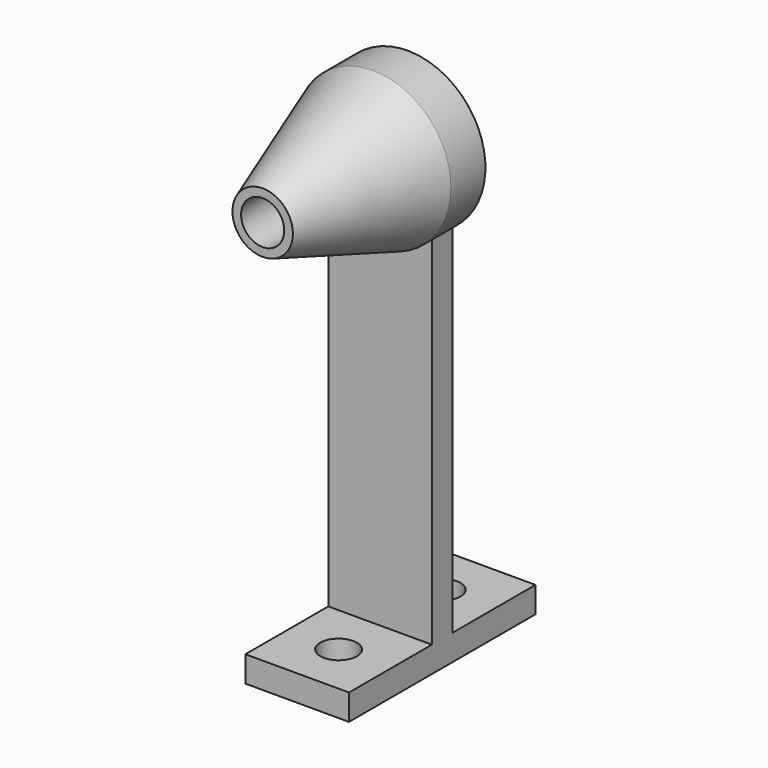
from build123d import *
from build123d import SkipClean  # not in build123d's __all__

# Parameters (mm, degrees)
F0_R      = 28.575
F2_R      = 11.1125
F4_R      = 7.9375
F5_DEPTH  = 50.8010001
F6_R      = 28.575
F6_R_2    = 7.9375
F7_DEPTH  = 15.875
F10_DEPTH = 9.525
F11_W     = 38.1
F11_H     = 85.725
F12_DEPTH = 9.525
F13_R     = 6.746875
F14_DEPTH = 9.526


# Not quite as in the source:
# - after a boolean that leaves OpenCascade's solid faulty, fix() repairs it


with BuildPart() as f3:
    # F0 (on Front) → F3 section 0
    with BuildSketch(Plane.XZ):
        Circle(F0_R)
    # F2 (on offset) → F3 section 1
    with BuildSketch(Plane.XZ.offset(50.8)):
        Circle(F2_R)
    loft()

    # F4 (on face) → F5 (cut, through all)
    with BuildSketch(Plane.XZ.offset(50.8)):
        Circle(F4_R)
    extrude(amount=-F5_DEPTH, mode=Mode.SUBTRACT)

    # F6 (on face) → F7 (join)
    with BuildSketch(Plane(origin=(0, 0, 0), x_dir=(-1, 0, 0), z_dir=(0, 1, 0))):
        Circle(F6_R)
        Circle(F6_R_2, mode=Mode.SUBTRACT)
    with SkipClean():  # cleaning this boolean's faces spoils the solid; the shape is the same uncleaned
        extrude(amount=F7_DEPTH)

    # F9 (on offset) → F10 (join)
    with BuildSketch(Plane.XZ.offset(-3.175)):
        with BuildLine():
            ThreePointArc((19.05, -21.2985474857), (0, -28.575), (-19.05, -21.2985474857))
            Line((-19.05, -21.2985474857), (-19.05, -152.4))
            Line((-19.05, -152.4), (19.05, -152.4))
            Line((19.05, -152.4), (19.05, -21.2985474857))
        make_face()
    extrude(amount=-F10_DEPTH)

    add(f3.part.fix(), mode=Mode.REPLACE)

    # F11 (on face) → F12 (join)
    with BuildSketch(Plane(origin=(0, 0, -152.4), x_dir=(1, 0, 0), z_dir=(0, 0, -1))):
        with Locations((0, -7.9375)):
            Rectangle(F11_W, F11_H)
    extrude(amount=F12_DEPTH)

    add(f3.part.fix(), mode=Mode.REPLACE)

    # F13 (on face) → F14 (cut, through all)
    with BuildSketch(Plane.XY.offset(-152.4)):
        with Locations((0, 31.75)):
            Circle(F13_R)
        with Locations((0, -15.875)):
            Circle(F13_R)
    extrude(amount=-F14_DEPTH, mode=Mode.SUBTRACT)


solid = f3.part
